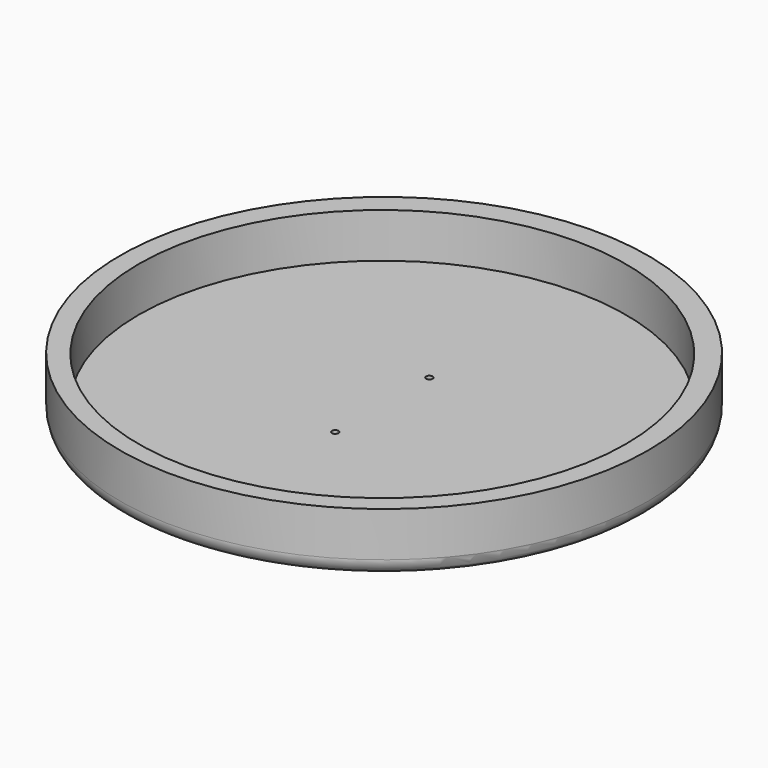
from build123d import *

# Parameters (mm, degrees)
F0_R     = 325
F1_DEPTH = 75
F2_R     = 300
F3_DEPTH = 55
F4_R     = 20
F6_DEPTH = 25


with BuildPart() as f1:
    # F0 (on Top) → F1 (new body)
    with BuildSketch(Plane.XY):
        with Locations((0, 2.7766637504)):
            Circle(F0_R)
    extrude(amount=F1_DEPTH)

    # F2 (on face) → F3 (cut)
    with BuildSketch(Plane.XY.offset(75)):
        Circle(F2_R)
    extrude(amount=-F3_DEPTH, mode=Mode.SUBTRACT)

    # F4
    f4_edges = [f1.edges().sort_by_distance(p)[0] for p in [
        (-325, 2.776664, 0),
    ]]
    fillet(f4_edges, radius=F4_R)

    # F5 (on face) → F6 (cut)
    with BuildSketch(Plane.XY.offset(20)):
        with BuildLine():
            ThreePointArc((-3.9984777127, 72.3896551724), (0, 68.5), (3.9984777127, 72.3896551724))
            ThreePointArc((3.9984777127, 72.3896551724), (0, 72.5), (-3.9984777127, 72.3896551724))
        make_face()
        with BuildLine():
            ThreePointArc((-3.9984777127, 72.3896551724), (0, 72.5), (3.9984777127, 72.3896551724))
            ThreePointArc((3.9984777127, 72.3896551724), (3.9996194101, 72.4448223362), (4, 72.5))
            ThreePointArc((4, 72.5), (-0.0551776638, 76.4996194101), (-3.9984777127, 72.3896551724))
        make_face()
        with BuildLine():
            ThreePointArc((4, -72.5), (3.9996194101, -72.4448223362), (3.9984777127, -72.3896551724))
            ThreePointArc((3.9984777127, -72.3896551724), (0, -72.5), (-3.9984777127, -72.3896551724))
            ThreePointArc((-3.9984777127, -72.3896551724), (-0.0551776638, -76.4996194101), (4, -72.5))
        make_face()
        with BuildLine():
            ThreePointArc((-3.9984777127, -72.3896551724), (0, -72.5), (3.9984777127, -72.3896551724))
            ThreePointArc((3.9984777127, -72.3896551724), (0, -68.5), (-3.9984777127, -72.3896551724))
        make_face()
    extrude(amount=-F6_DEPTH, mode=Mode.SUBTRACT)


solid = f1.part
